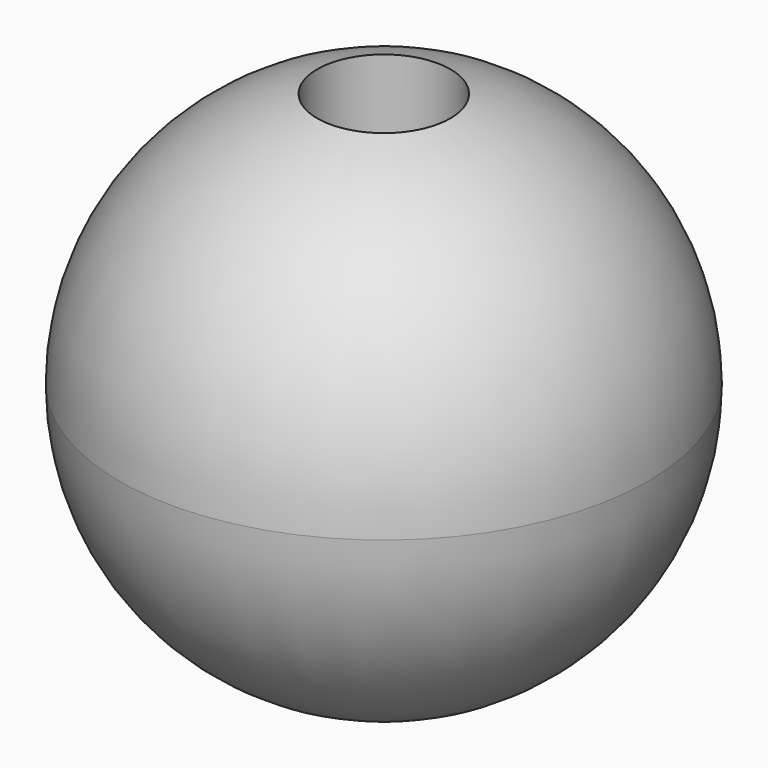
from build123d import *

# Parameters (mm, degrees)
F0_R     = 12.7
F1_DEPTH = 25.4
F2_R     = 12.69999
F3_R     = 3.2007546804
F4_DEPTH = 25.401


# Not quite as in the source:
# - a fillet or chamfer is up to 0.001 mm smaller than in the source, because OpenCascade refuses the exact size


with BuildPart() as f1:
    # F0 (on Top) → F1 (new body)
    with BuildSketch(Plane.XY):
        Circle(F0_R)
    extrude(amount=F1_DEPTH)

    # F2 (radius 12.7 in the source; OpenCascade refuses exactly that, so slightly less here)
    f2_edges = [f1.edges().sort_by_distance(p)[0] for p in [
        (-12.7, 0, 25.4),
        (-12.7, 0, 0),
    ]]
    fillet(f2_edges, radius=F2_R)

    # F3 (on Top) → F4 (cut, through all)
    with BuildSketch(Plane.XY):
        Circle(F3_R)
    extrude(amount=F4_DEPTH, mode=Mode.SUBTRACT)


solid = f1.part
